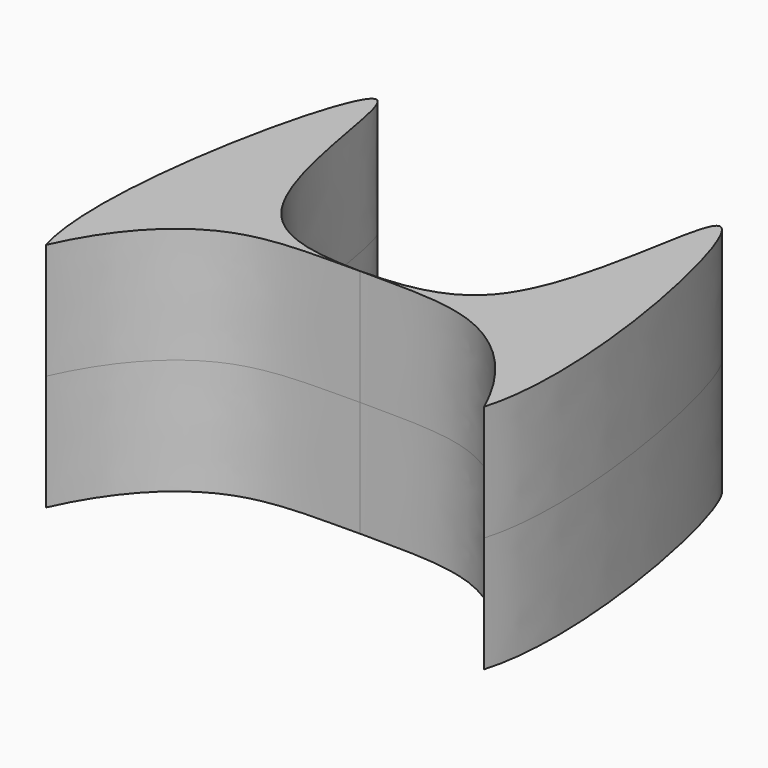
from build123d import *

# Parameters (mm, degrees)
F1_DEPTH = 25.4
F2_DEPTH = 25.4


# Not quite as in the source:
# - a pattern or mirror of a feature is missing from the dataset's text; its kind, count and spacing are read off the source's solid


with BuildPart() as f1:
    # F0 (on Top) → F1 (new body)
    with BuildSketch(Plane.XY):
        with BuildLine():
            add(Edge.make_bspline(
                [(0, 17.9789804723), (-9.3970661986, 18.1508080752), (-34.1681733574, 20.9558499948), (-33.7341512053, 111.0583110271), (-54.7725797856, 13.6405870148), (-48.129248964, -8.0604708915)],
                knots=[0.2144038498, 0.2144038498, 0.2144038498, 0.2144038498, 0.2877075932, 0.4213604409, 0.5844153219, 0.5844153219, 0.5844153219, 0.5844153219], degree=3))
            add(Edge.make_bspline(
                [(-48.129248964, -8.0604708915), (-43.214344744, 2.9421106636), (-29.6383542096, 19.0452197015), (-8.5887730826, 17.8219327024), (0, 17.9789804723)],
                knots=[0.0595860268, 0.0595860268, 0.0595860268, 0.0595860268, 0.1474053628, 0.2144038498, 0.2144038498, 0.2144038498, 0.2144038498], degree=3))
        make_face()
    extrude(amount=F1_DEPTH)


with BuildPart() as f1b:
    # F0 (on Top) → F1, piece 2 (new body)
    with BuildSketch(Plane.XY):
        with BuildLine():
            add(Edge.make_bspline(
                [(0, 17.9789804723), (9.3970661986, 18.1508080752), (34.1681733574, 20.9558499948), (33.7341512054, 111.0583110203), (54.7725797817, 13.6405870331), (48.1292489674, -8.0604708804)],
                knots=[0.2144038498, 0.2144038498, 0.2144038498, 0.2144038498, 0.2877075932, 0.4213604409, 0.5844153219, 0.5844153219, 0.5844153219, 0.5844153219], degree=3))
            add(Edge.make_bspline(
                [(48.129248959, -8.0604708805), (43.2143447389, 2.9421106697), (29.6383542056, 19.0452197013), (8.5887730826, 17.8219327024), (0, 17.9789804723)],
                knots=[0.0595860268, 0.0595860268, 0.0595860268, 0.0595860268, 0.1474053628, 0.2144038498, 0.2144038498, 0.2144038498, 0.2144038498], degree=3))
        make_face()
    extrude(amount=F1_DEPTH)


with BuildPart() as f1_copies_1:
    # F1_copies: instance of F1
    add(f1.part.mirror(Plane(origin=(0, 0, 0), x_dir=(-1, 0, 0), z_dir=(0, 0, -1))))


with BuildPart() as f2:
    # F2 (new): faces of the model
    f2_faces = [f1b.part.faces().sort_by_distance(p)[0] for p in [
        (37.8664105419, 29.1812237323, 0),
        (37.8664105419, 29.1812237323, 0),
    ]]
    extrude(f2_faces, amount=F2_DEPTH)


solid = Compound([f1.part, f1b.part, f1_copies_1.part, f2.part])
